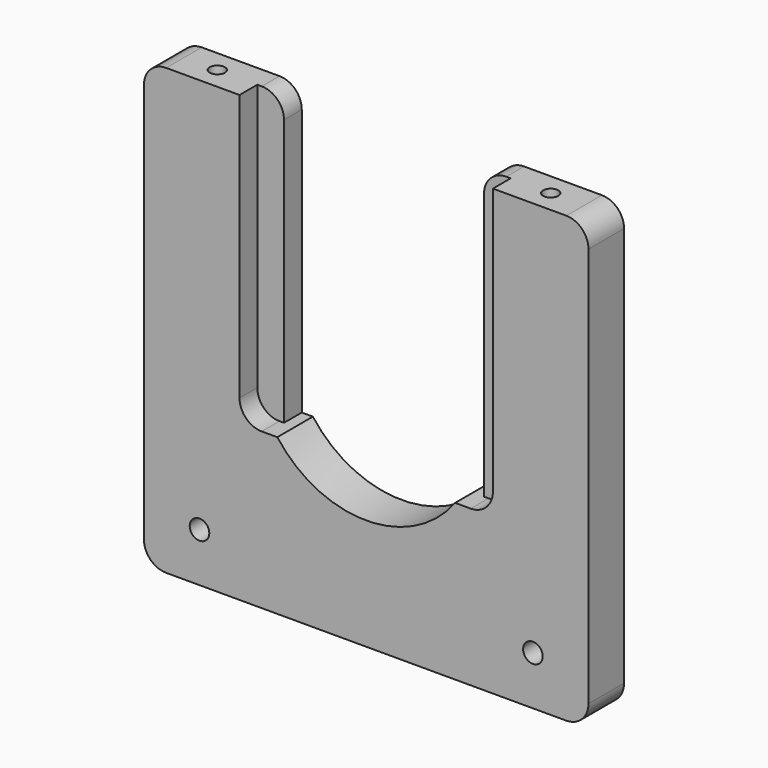
from build123d import *

# Parameters (mm, degrees)
F0_W      = 200
F0_H      = 200
F1_DEPTH  = 10
F2_R      = 15
F3_DEPTH  = 20.001
F5_D      = 8.8
F7_DEPTH  = 20.001
F8_W      = 12
F8_H      = 130
F9_DEPTH  = 10
F10_R     = 10
F13_D     = 6.8
F13_DEPTH = 19.25
F13_TIP   = 2.0429261047


# Not quite as in the source:
# - two fillets or chamfers of one size are made in one step
# - a feature names something its author has since deleted; it is built from what else it names


with BuildPart() as f1:
    # F0 (on Front) → F1 (new body, symmetric)
    with BuildSketch(Plane.XZ):
        Rectangle(F0_W, F0_H)
    extrude(amount=F1_DEPTH, both=True)

    # F2 (on face) → F3 (cut, through all)
    with BuildSketch(Plane.XZ.offset(10)):
        Circle(F2_R)
    extrude(amount=-F3_DEPTH, mode=Mode.SUBTRACT)

    # F5 (through all)
    with Locations(Plane.XZ.offset(10)):
        with Locations((-75, -78), (75, -78)):
            Hole(F5_D / 2)

    # F6 (on face) → F7 (cut, through all)
    with BuildSketch(Plane.XZ.offset(10)):
        with BuildLine():
            Line((45, 100), (-45, 100))
            Line((-45, 100), (-45, -30))
            Line((-45, -30), (-40, -30))
            ThreePointArc((-40, -30), (0, -50), (40, -30))
            Line((40, -30), (45, -30))
            Line((45, -30), (45, 100))
        make_face()
    extrude(amount=-F7_DEPTH, mode=Mode.SUBTRACT)

    # F8 (on face) → F9 (cut)
    with BuildSketch(Plane.XZ.offset(10)):
        with Locations((-51, 35)):
            Rectangle(F8_W, F8_H)
        with Locations((51, 35)):
            Rectangle(F8_W, F8_H)
    extrude(amount=-F9_DEPTH, mode=Mode.SUBTRACT)

    # F10
    f10_edges = [f1.edges().sort_by_distance(p)[0] for p in [
        (-100, 0, 100),
        (-45, 5, 100),
        (45, 5, 100),
        (100, 0, 100),
        (100, 0, -100),
        (-100, 0, -100),
        (-57, -5, -30),
        (57, -5, -30),
    ]]
    fillet(f10_edges, radius=F10_R)

    # F13
    with Locations(Plane.XY.offset(100)):
        with Locations((-75, 0), (75, 0)):
            Hole(F13_D / 2, depth=F13_DEPTH)
            with Locations((0, 0, -(F13_DEPTH + F13_TIP / 2))):  # 118° drill point
                Cone(0, F13_D / 2, F13_TIP, mode=Mode.SUBTRACT)


solid = f1.part
